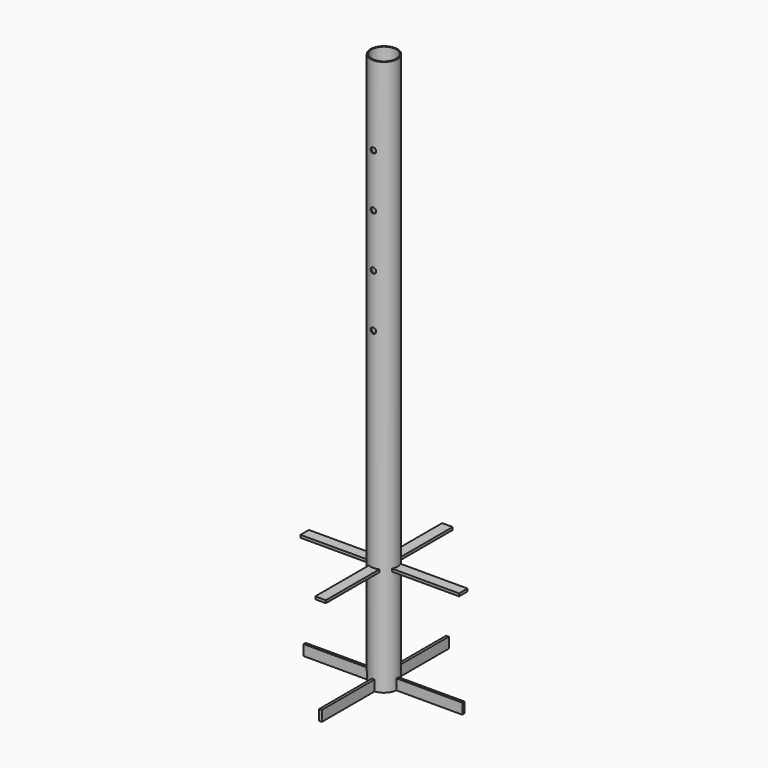
from build123d import *

# Parameters (mm, degrees)
F0_R            = 25.5
F0_R_2          = 23.5
F1_DEPTH        = 1050
F3_W            = 5
F3_H            = 20
F3_W_2          = 20
F3_H_2          = 5
F4_COPIES_COUNT = 4
F5_R            = 5.25
F6_DEPTH        = 150.001
F6_DEPTH_BACK   = 150.001


# Not quite as in the source:
# - a pattern or mirror of a feature is missing from the dataset's text; its kind, count and spacing are read off the source's solid


with BuildPart() as f1:
    # F0 (on Top) → F1 (new body)
    with BuildSketch(Plane.XY):
        Circle(F0_R)
        Circle(F0_R_2, mode=Mode.SUBTRACT)
    extrude(amount=F1_DEPTH)

    # F3 (on offset) → F4 (join, up to the next surface of F1)
    with BuildSketch(Plane.YZ.offset(150)):
        with Locations((0, 10)):
            Rectangle(F3_W, F3_H)
        with Locations((0, 202.5)):
            Rectangle(F3_W_2, F3_H_2)
    f4 = extrude(until=Until.NEXT, dir=(-1, 0, 0))

    # F4_copies: F4 ×4 about axis
    f4_copies_axis = Axis((0, 0, 0), (0, 0, 1))
    for i in range(1, F4_COPIES_COUNT):
        add(f4.rotate(f4_copies_axis, i * 360 / F4_COPIES_COUNT))

    # F5 (on Front) → F6 (cut, two sides)
    with BuildSketch(Plane.XZ) as f6_sk:
        with Locations((0, 600)):
            Circle(F5_R)
        with Locations((0, 700)):
            Circle(F5_R)
        with Locations((0, 800)):
            Circle(F5_R)
        with Locations((0, 900)):
            Circle(F5_R)
    extrude(amount=-F6_DEPTH, mode=Mode.SUBTRACT)
    extrude(f6_sk.sketch, amount=F6_DEPTH_BACK, mode=Mode.SUBTRACT)


solid = f1.part
